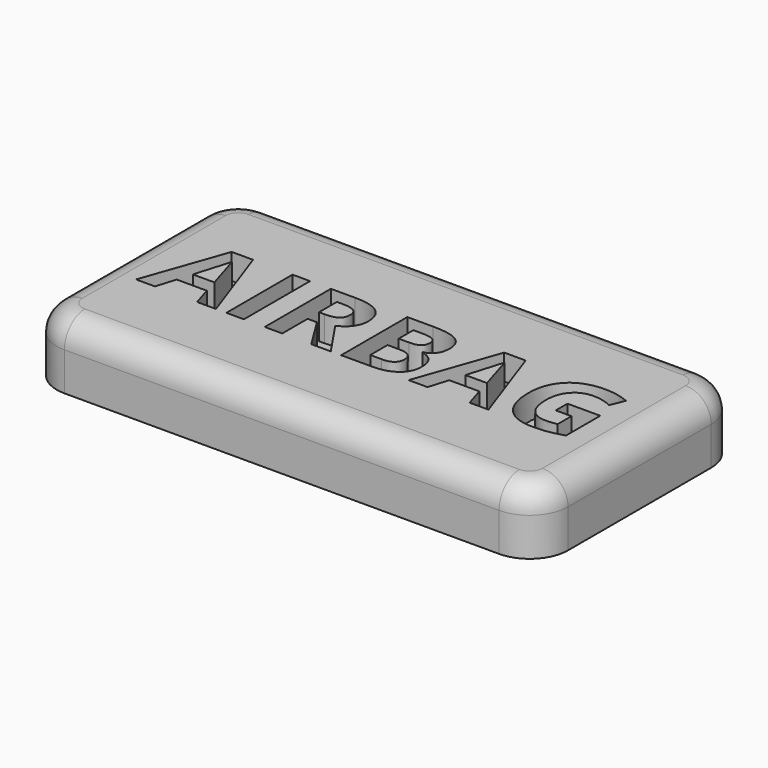
from build123d import *

# Parameters (mm, degrees)
F0_W         = 0.6815827911
F0_H         = 5.8646926039
F0_TEXT_SIZE = 8.2149338291
F1_DEPTH     = 5
F2_TEXT_SIZE = 9.0617582143
F3_DEPTH     = 2
F4_R         = 2


# Not quite as in the source:
# - Text() gives the source's letters only with a copy of the font that has no kerning and outlines rounded to 1/6400 em; it was checked with that copy


with BuildPart() as f1:
    # F0 (on Top) → F1 (new body)
    with BuildSketch(Plane.XY):
        with BuildLine():
            Line((17.1850156114, 8.8056281811), (-16.8149843886, 8.8056281811))
            ThreePointArc((-16.8149843886, 8.8056281811), (-18.9363047322, 7.9269485247), (-19.8149843886, 5.8056281811))
            Line((-19.8149843886, 5.8056281811), (-19.8149843886, -8.1943718189))
            ThreePointArc((-19.8149843886, -8.1943718189), (-18.9363047322, -10.3156921624), (-16.8149843886, -11.1943718189))
            Line((-16.8149843886, -11.1943718189), (17.1850156114, -11.1943718189))
            ThreePointArc((17.1850156114, -11.1943718189), (19.3063359549, -10.3156921624), (20.1850156114, -8.1943718189))
            Line((20.1850156114, -8.1943718189), (20.1850156114, 5.8056281811))
            ThreePointArc((20.1850156114, 5.8056281811), (19.3063359549, 7.9269485247), (17.1850156114, 8.8056281811))
        make_face()
        Polygon((-9.1164715749, -4.1091241758), (-9.8224424509, -4.1091241758), (-10.5528014116, -2.2440774799), (-12.9030426368, -2.2440774799), (-13.6244165136, -4.1091241758), (-14.3149843886, -4.1091241758), (-11.9968327488, 1.7799565129), (-11.4230709641, 1.7799565129), align=None, mode=Mode.SUBTRACT)
        with Locations((-7.9695897974, -1.1767778738)):
            Rectangle(F0_W, F0_H, mode=Mode.SUBTRACT)
        with BuildLine():
            Line((-4.1143470231, -1.6703156953), (-5.338885597, -1.6703156953))
            Line((-5.338885597, -1.6703156953), (-5.338885597, -4.1091241758))
            Line((-5.338885597, -4.1091241758), (-6.0204683881, -4.1091241758))
            Line((-6.0204683881, -4.1091241758), (-6.0204683881, 1.7555684281))
            Line((-6.0204683881, 1.7555684281), (-4.4121383744, 1.7555684281))
            add(Edge.make_bspline(
                [(-4.4121383744, 1.7555684281), (-3.3326447259, 1.7555684281), (-2.8172859865, 1.3422545698)],
                knots=[0, 0, 0, 1, 1, 1], degree=2))
            add(Edge.make_bspline(
                [(-2.8172859865, 1.3422545698), (-2.3019272471, 0.9289407116), (-2.3019272471, 0.0984622448)],
                knots=[0, 0, 0, 1, 1, 1], degree=2))
            add(Edge.make_bspline(
                [(-2.3019272471, 0.0984622448), (-2.3019272471, -1.0644643254), (-3.4815404016, -1.4739274334)],
                knots=[0, 0, 0, 1, 1, 1], degree=2))
            Line((-3.4815404016, -1.4739274334), (-1.8886133888, -4.1091241758))
            Line((-1.8886133888, -4.1091241758), (-2.6947037708, -4.1091241758))
            Line((-2.6947037708, -4.1091241758), (-4.1143470231, -1.6703156953))
        make_face(mode=Mode.SUBTRACT)
        with BuildLine():
            Line((-0.942612415, -4.1091241758), (-0.942612415, 1.7555684281))
            Line((-0.942612415, 1.7555684281), (0.7144937683, 1.7555684281))
            add(Edge.make_bspline(
                [(0.7144937683, 1.7555684281), (1.8812710887, 1.7555684281), (2.4030477452, 1.4064337404)],
                knots=[0, 0, 0, 1, 1, 1], degree=2))
            add(Edge.make_bspline(
                [(2.4030477452, 1.4064337404), (2.9248244017, 1.0572990526), (2.9248244017, 0.3038355905)],
                knots=[0, 0, 0, 1, 1, 1], degree=2))
            add(Edge.make_bspline(
                [(2.9248244017, 0.3038355905), (2.9248244017, -0.2185828577), (2.6340927591, -0.5574488781)],
                knots=[0, 0, 0, 1, 1, 1], degree=2))
            add(Edge.make_bspline(
                [(2.6340927591, -0.5574488781), (2.3433611166, -0.8963148986), (1.7850023329, -0.9964344046)],
                knots=[0, 0, 0, 1, 1, 1], degree=2))
            Line((1.7850023329, -0.9964344046), (1.7850023329, -1.0362254904))
            add(Edge.make_bspline(
                [(1.7850023329, -1.0362254904), (3.1212126635, -1.2647033375), (3.1212126635, -2.4404657418)],
                knots=[0, 0, 0, 1, 1, 1], degree=2))
            add(Edge.make_bspline(
                [(3.1212126635, -2.4404657418), (3.1212126635, -3.2260187892), (2.5898091315, -3.6675714825)],
                knots=[0, 0, 0, 1, 1, 1], degree=2))
            add(Edge.make_bspline(
                [(2.5898091315, -3.6675714825), (2.0584055994, -4.1091241758), (1.1034195418, -4.1091241758)],
                knots=[0, 0, 0, 1, 1, 1], degree=2))
            Line((1.1034195418, -4.1091241758), (-0.942612415, -4.1091241758))
        make_face(mode=Mode.SUBTRACT)
        Polygon((8.7728304212, -4.1091241758), (8.0668595453, -4.1091241758), (7.3365005846, -2.2440774799), (4.9862593594, -2.2440774799), (4.2648854825, -4.1091241758), (3.5743176075, -4.1091241758), (5.8924692474, 1.7799565129), (6.4662310321, 1.7799565129), align=None, mode=Mode.SUBTRACT)
        with BuildLine():
            Line((12.1589234589, -1.6459276105), (12.1589234589, -1.0362254904))
            Line((12.1589234589, -1.0362254904), (14.1523284959, -1.0362254904))
            Line((14.1523284959, -1.0362254904), (14.1523284959, -3.8883478291))
            add(Edge.make_bspline(
                [(14.1523284959, -3.8883478291), (13.6863877178, -4.0372435048), (13.2050439387, -4.1136167177)],
                knots=[0, 0, 0, 1, 1, 1], degree=2))
            add(Edge.make_bspline(
                [(13.2050439387, -4.1136167177), (12.7237001597, -4.1899899307), (12.0896099547, -4.1899899307)],
                knots=[0, 0, 0, 1, 1, 1], degree=2))
            add(Edge.make_bspline(
                [(12.0896099547, -4.1899899307), (10.7585339577, -4.1899899307), (10.0166227463, -3.3973771745)],
                knots=[0, 0, 0, 1, 1, 1], degree=2))
            add(Edge.make_bspline(
                [(10.0166227463, -3.3973771745), (9.2747115349, -2.6047644184), (9.2747115349, -1.1774196656)],
                knots=[0, 0, 0, 1, 1, 1], degree=2))
            add(Edge.make_bspline(
                [(9.2747115349, -1.1774196656), (9.2747115349, -0.2622246937), (9.6418163904, 0.4257760145)],
                knots=[0, 0, 0, 1, 1, 1], degree=2))
            add(Edge.make_bspline(
                [(9.6418163904, 0.4257760145), (10.0089212458, 1.1137767227), (10.6988473291, 1.4763890363)],
                knots=[0, 0, 0, 1, 1, 1], degree=2))
            add(Edge.make_bspline(
                [(10.6988473291, 1.4763890363), (11.3887734124, 1.8390013498), (12.3142370516, 1.8390013498)],
                knots=[0, 0, 0, 1, 1, 1], degree=2))
            add(Edge.make_bspline(
                [(12.3142370516, 1.8390013498), (13.2538201083, 1.8390013498), (14.0637612405, 1.4950009957)],
                knots=[0, 0, 0, 1, 1, 1], degree=2))
            Line((14.0637612405, 1.4950009957), (13.7993430579, 0.8930003761))
            add(Edge.make_bspline(
                [(13.7993430579, 0.8930003761), (13.0048049266, 1.2292992297), (12.2705952157, 1.2292992297)],
                knots=[0, 0, 0, 1, 1, 1], degree=2))
            add(Edge.make_bspline(
                [(12.2705952157, 1.2292992297), (11.2000866511, 1.2292992297), (10.5980860314, 0.5920000662)],
                knots=[0, 0, 0, 1, 1, 1], degree=2))
            add(Edge.make_bspline(
                [(10.5980860314, 0.5920000662), (9.9960854117, -0.0452990972), (9.9960854117, -1.1774196656)],
                knots=[0, 0, 0, 1, 1, 1], degree=2))
            add(Edge.make_bspline(
                [(9.9960854117, -1.1774196656), (9.9960854117, -2.3647343205), (10.5756233217, -2.9782871909)],
                knots=[0, 0, 0, 1, 1, 1], degree=2))
            add(Edge.make_bspline(
                [(10.5756233217, -2.9782871909), (11.1551612317, -3.5918400613), (12.2782967161, -3.5918400613)],
                knots=[0, 0, 0, 1, 1, 1], degree=2))
            add(Edge.make_bspline(
                [(12.2782967161, -3.5918400613), (12.8879988362, -3.5918400613), (13.4694621213, -3.4506458861)],
                knots=[0, 0, 0, 1, 1, 1], degree=2))
            Line((13.4694621213, -3.4506458861), (13.4694621213, -1.6459276105))
            Line((13.4694621213, -1.6459276105), (12.1589234589, -1.6459276105))
        make_face(mode=Mode.SUBTRACT)
        with BuildLine():
            Line((0.9070312799, -1.3327332583), (-0.2610296239, -1.3327332583))
            Line((-0.2610296239, -1.3327332583), (-0.2610296239, -3.5276608907))
            Line((-0.2610296239, -3.5276608907), (0.96350895, -3.5276608907))
            add(Edge.make_bspline(
                [(0.96350895, -3.5276608907), (1.6733305762, -3.5276608907), (2.0320921395, -3.2529740408)],
                knots=[0, 0, 0, 1, 1, 1], degree=2))
            add(Edge.make_bspline(
                [(2.0320921395, -3.2529740408), (2.3908537028, -2.9782871909), (2.3908537028, -2.3916895722)],
                knots=[0, 0, 0, 1, 1, 1], degree=2))
            add(Edge.make_bspline(
                [(2.3908537028, -2.3916895722), (2.3908537028, -1.8461666226), (2.0237488473, -1.5894499404)],
                knots=[0, 0, 0, 1, 1, 1], degree=2))
            add(Edge.make_bspline(
                [(2.0237488473, -1.5894499404), (1.6566439918, -1.3327332583), (0.9070312799, -1.3327332583)],
                knots=[0, 0, 0, 1, 1, 1], degree=2))
        make_face()
        with BuildLine():
            Line((-5.338885597, 1.1574185587), (-5.338885597, -1.08500166))
            Line((-5.338885597, -1.08500166), (-4.4031532905, -1.08500166))
            add(Edge.make_bspline(
                [(-4.4031532905, -1.08500166), (-3.6817794137, -1.08500166), (-3.3448387683, -0.7981207677)],
                knots=[0, 0, 0, 1, 1, 1], degree=2))
            add(Edge.make_bspline(
                [(-3.3448387683, -0.7981207677), (-3.007898123, -0.5112398754), (-3.007898123, 0.0625219093)],
                knots=[0, 0, 0, 1, 1, 1], degree=2))
            add(Edge.make_bspline(
                [(-3.007898123, 0.0625219093), (-3.007898123, 0.6439851944), (-3.3506148937, 0.9007018765)],
                knots=[0, 0, 0, 1, 1, 1], degree=2))
            add(Edge.make_bspline(
                [(-3.3506148937, 0.9007018765), (-3.6933316644, 1.1574185587), (-4.4519294601, 1.1574185587)],
                knots=[0, 0, 0, 1, 1, 1], degree=2))
            Line((-4.4519294601, 1.1574185587), (-5.338885597, 1.1574185587))
        make_face()
        with BuildLine():
            Line((-0.2610296239, 1.1651200591), (-0.2610296239, -0.7551207234))
            Line((-0.2610296239, -0.7551207234), (0.8621058605, -0.7551207234))
            add(Edge.make_bspline(
                [(0.8621058605, -0.7551207234), (1.5847633208, -0.7551207234), (1.9018084233, -0.5285682514)],
                knots=[0, 0, 0, 1, 1, 1], degree=2))
            add(Edge.make_bspline(
                [(1.9018084233, -0.5285682514), (2.2188535257, -0.3020157794), (2.2188535257, 0.2345220863)],
                knots=[0, 0, 0, 1, 1, 1], degree=2))
            add(Edge.make_bspline(
                [(2.2188535257, 0.2345220863), (2.2188535257, 0.7287016995), (1.8658680878, 0.9469108793)],
                knots=[0, 0, 0, 1, 1, 1], degree=2))
            add(Edge.make_bspline(
                [(1.8658680878, 0.9469108793), (1.5128826498, 1.1651200591), (0.7427326033, 1.1651200591)],
                knots=[0, 0, 0, 1, 1, 1], degree=2))
            Line((0.7427326033, 1.1651200591), (-0.2610296239, 1.1651200591))
        make_face()
        with Locations((-14.3149843886, -4.1091241758)):
            Text('AIRBAG', F0_TEXT_SIZE, font='Open Sans', text_align=(TextAlign.LEFT, TextAlign.BOTTOM))
        with BuildLine():
            Line((-12.6617289556, -1.6305246096), (-10.7645926744, -1.6305246096))
            Line((-10.7645926744, -1.6305246096), (-11.4474590489, 0.1870295001))
            add(Edge.make_bspline(
                [(-11.4474590489, 0.1870295001), (-11.5796681403, 0.5323134376), (-11.719578732, 1.0329109678)],
                knots=[0, 0, 0, 1, 1, 1], degree=2))
            add(Edge.make_bspline(
                [(-11.719578732, 1.0329109678), (-11.8081459874, 0.6478359446), (-11.972444664, 0.1870295001)],
                knots=[0, 0, 0, 1, 1, 1], degree=2))
            Line((-11.972444664, 0.1870295001), (-12.6617289556, -1.6305246096))
        make_face()
        with BuildLine():
            Line((5.2275730406, -1.6305246096), (7.1247093218, -1.6305246096))
            Line((7.1247093218, -1.6305246096), (6.4418429473, 0.1870295001))
            add(Edge.make_bspline(
                [(6.4418429473, 0.1870295001), (6.3096338559, 0.5323134376), (6.1697232642, 1.0329109678)],
                knots=[0, 0, 0, 1, 1, 1], degree=2))
            add(Edge.make_bspline(
                [(6.1697232642, 1.0329109678), (6.0811560088, 0.6478359446), (5.9168573322, 0.1870295001)],
                knots=[0, 0, 0, 1, 1, 1], degree=2))
            Line((5.9168573322, 0.1870295001), (5.2275730406, -1.6305246096))
        make_face()
    extrude(amount=F1_DEPTH)

    # F2 (on face) → F3 (cut)
    with BuildSketch(Plane.XY.offset(5)):
        with Locations((-16.8149843886, -4.1943718189)):
            Text('AIRBAG', F2_TEXT_SIZE, font='Open Sans', font_style=FontStyle.BOLD, text_align=(TextAlign.LEFT, TextAlign.BOTTOM))
    extrude(amount=-F3_DEPTH, mode=Mode.SUBTRACT)

    # F4
    f4_edges = [f1.edges().sort_by_distance(p)[0] for p in [
        (-19.814984, -1.194372, 5),
        (-18.936305, -10.315692, 5),
        (0.185016, -11.194372, 5),
        (19.306336, -10.315692, 5),
        (20.185016, -1.194372, 5),
        (19.306336, 7.926949, 5),
        (0.185016, 8.805628, 5),
        (-18.936305, 7.926949, 5),
    ]]
    fillet(f4_edges, radius=F4_R)


solid = f1.part
